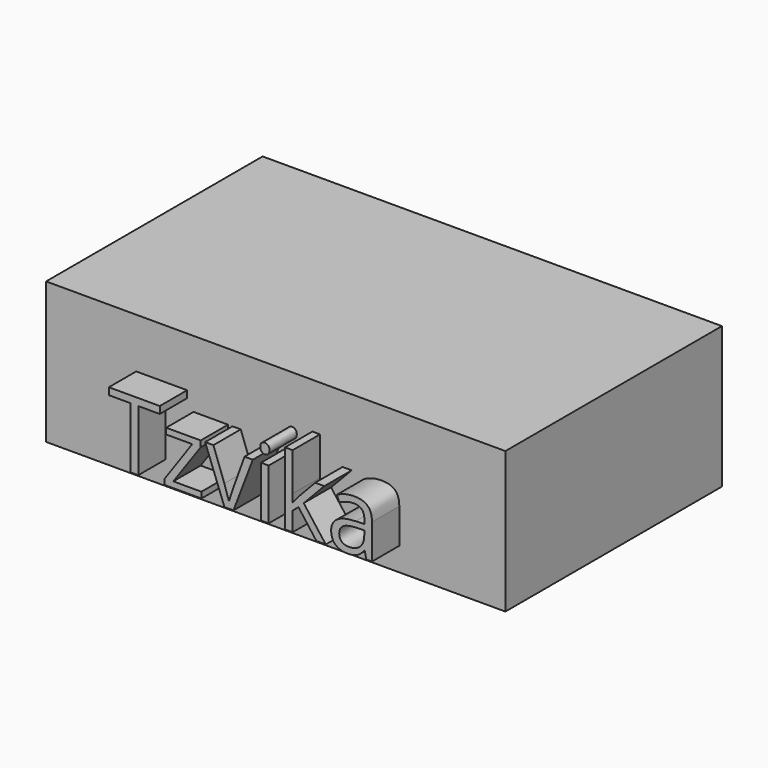
from build123d import *

# Parameters (mm, degrees)
F0_W         = 102.3789532483
F0_H         = 60.3284239769
F1_DEPTH     = 31.496
F4_TEXT_SIZE = 21.2003399308
F5_DEPTH     = 7.62


# Not quite as in the source:
# - the program builds the solid bodies; features that only make, move or delete a surface that nothing else refers to are left out
# - Text() gives the source's letters only with a copy of the font that has no kerning and outlines rounded to 1/6400 em; it was checked with that copy


with BuildPart() as f1:
    # F0 (on Top) → F1 (new body)
    with BuildSketch(Plane.XY):
        with Locations((3.0246879905, 0.0163782388)):
            Rectangle(F0_W, F0_H)
    extrude(amount=F1_DEPTH)

    # F4 (on face) → F5 (join)
    with BuildSketch(Plane.XZ.offset(30.1478337497)):
        with Locations((-28.2594774617, 5.2289552987)):
            Text('Tzvika', F4_TEXT_SIZE, font='Open Sans', text_align=(TextAlign.LEFT, TextAlign.BOTTOM))
    extrude(amount=F5_DEPTH)


solid = f1.part
